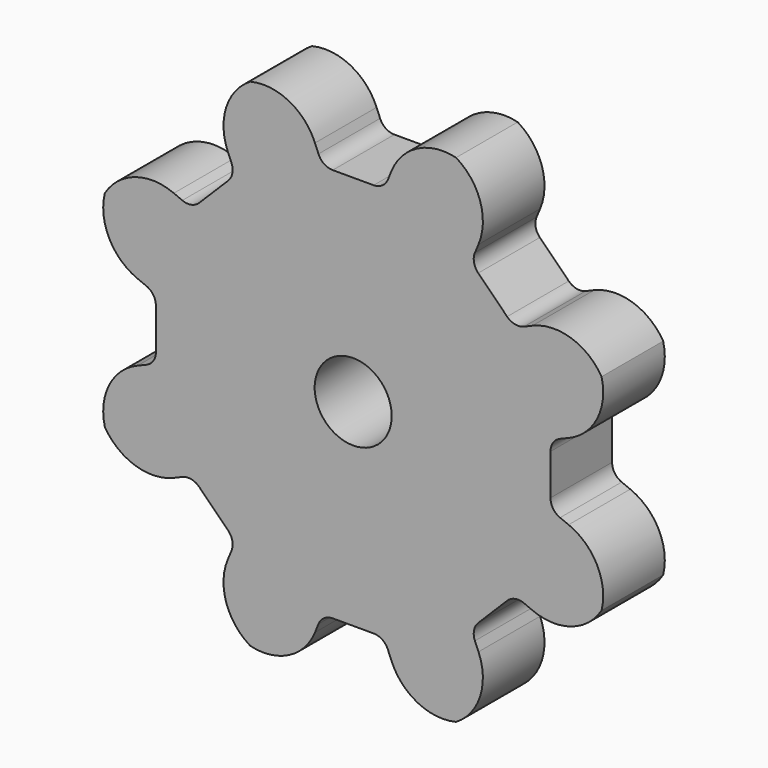
from build123d import *

# Parameters (mm, degrees)
F0_W            = 6.35
F0_H            = 22.225
F3_DEPTH        = 6.35
F3_COPIES_COUNT = 8
F4_T1_DEPTH     = 30.2839966419
F4_T3_DEPTH     = 30.283996606
F5_R            = 3.175
F6_DEPTH        = 6.35


# Not quite as in the source:
# - a fillet or chamfer that OpenCascade refuses, or shapes differently, is made with other operations: its cross-section is extruded or revolved along the edge and cut away or added
# - a pattern or mirror of a feature is missing from the dataset's text; its kind, count and spacing are read off the source's solid


with BuildPart() as f1:
    # F0 (on Right) → F1 (revolve)
    with BuildSketch(Plane.YZ):
        with Locations((3.175, 33.3375)):
            Rectangle(F0_W, F0_H)
    revolve(axis=Axis((0, 3.175, 22.225), (0, 1, 0)))

    # F2 (on Front) → F3 (cut)
    with BuildSketch(Plane.XZ):
        with BuildLine():
            Line((-1.59e-08, 38.4876703219), (-1.59e-08, 44.3230155219))
            Line((-1.59e-08, 44.3230155219), (-1.59e-08, 44.457260554))
            Line((-1.59e-08, 44.457260554), (-4.9701853855, 44.457260554))
            Line((-4.9701853855, 44.457260554), (-4.9155350159, 44.3230155219))
            Line((-4.9155350159, 44.3230155219), (-2.8620721488, 39.2788192947))
            ThreePointArc((-2.8620721488, 39.2788192947), (-2.3945935663, 38.7038580036), (-1.6858061527, 38.4876703219))
            Line((-1.6858061527, 38.4876703219), (-1.59e-08, 38.4876703219))
        make_face()
        with BuildLine():
            Line((-1.59e-08, 44.457260554), (-1.59e-08, 44.3230155219))
            Line((-1.59e-08, 44.3230155219), (-1.59e-08, 38.4876703219))
            Line((-1.59e-08, 38.4876703219), (1.6858061209, 38.4876703219))
            ThreePointArc((1.6858061209, 38.4876703219), (2.3945935345, 38.7038580036), (2.8620721171, 39.2788192947))
            Line((2.8620721171, 39.2788192947), (4.9155349841, 44.3230155219))
            Line((4.9155349841, 44.3230155219), (4.9701853538, 44.457260554))
            Line((4.9701853538, 44.457260554), (-1.59e-08, 44.457260554))
        make_face()
    f3 = extrude(amount=-F3_DEPTH, mode=Mode.SUBTRACT)

    # F3_copies: F3 ×8 about axis
    f3_copies_axis = Axis((0, 0, 22.225), (0, 1, 0))
    for i in range(1, F3_COPIES_COUNT):
        add(f3.rotate(f3_copies_axis, i * 360 / F3_COPIES_COUNT), mode=Mode.SUBTRACT)

    # F4: fillet of radius 4.572 on 16 edges, made by hand

    # F4_s2 → F4_t1 (cut)
    with BuildSketch(Plane.XZ.offset(-18.3169983209)):
        with BuildLine():
            ThreePointArc((-3.1489730441, 39.9835724397), (-5.703273274, 42.5117575675), (-9.2958119446, 42.4125829482))
            ThreePointArc((-9.2958119446, 42.4125829482), (-7.0677616426, 43.2962451071), (-4.757507246, 43.934830718))
            Line((-4.757507246, 43.934830718), (-3.1489730441, 39.9835724397))
        make_face()
        with BuildLine():
            ThreePointArc((-10.330546803, 7.4411328104), (-10.3120806372, 3.8472729487), (-7.7016451357, 1.3770915389))
            ThreePointArc((-7.7016451357, 1.3770915389), (-9.901958118, 2.3277175114), (-11.9871028839, 3.5097658457))
            Line((-11.9871028839, 3.5097658457), (-10.330546803, 7.4411328104))
        make_face()
        with BuildLine():
            ThreePointArc((3.1489730441, 4.4664275603), (5.703273274, 1.9382424325), (9.2958119446, 2.0374170518))
            ThreePointArc((9.2958119446, 2.0374170518), (7.0677616426, 1.1537548929), (4.757507246, 0.515169282))
            Line((4.757507246, 0.515169282), (3.1489730441, 4.4664275603))
        make_face()
        with BuildLine():
            ThreePointArc((14.7838671896, 11.894453197), (18.3777270513, 11.9129193628), (20.8479084611, 14.5233548643))
            ThreePointArc((20.8479084611, 14.5233548643), (19.8972824886, 12.323041882), (18.7152341543, 10.2378971161))
            Line((18.7152341543, 10.2378971161), (14.7838671896, 11.894453197))
        make_face()
        with BuildLine():
            ThreePointArc((17.7585724397, 25.3739730441), (20.2867575675, 27.928273274), (20.1875829482, 31.5208119446))
            ThreePointArc((20.1875829482, 31.5208119446), (21.0712451071, 29.2927616426), (21.709830718, 26.982507246))
            Line((21.709830718, 26.982507246), (17.7585724397, 25.3739730441))
        make_face()
        with BuildLine():
            ThreePointArc((10.330546803, 37.0088671896), (10.3120806372, 40.6027270513), (7.7016451357, 43.0729084611))
            ThreePointArc((7.7016451357, 43.0729084611), (9.901958118, 42.1222824886), (11.9871028839, 40.9402341543))
            Line((11.9871028839, 40.9402341543), (10.330546803, 37.0088671896))
        make_face()
        with BuildLine():
            ThreePointArc((-14.7838671896, 32.555546803), (-18.3777270513, 32.5370806372), (-20.8479084611, 29.9266451357))
            ThreePointArc((-20.8479084611, 29.9266451357), (-19.8972824886, 32.126958118), (-18.7152341543, 34.2121028839))
            Line((-18.7152341543, 34.2121028839), (-14.7838671896, 32.555546803))
        make_face()
        with BuildLine():
            ThreePointArc((-17.7585724397, 19.0760269559), (-20.2867575675, 16.521726726), (-20.1875829482, 12.9291880554))
            ThreePointArc((-20.1875829482, 12.9291880554), (-21.0712451071, 15.1572383574), (-21.709830718, 17.467492754))
            Line((-21.709830718, 17.467492754), (-17.7585724397, 19.0760269559))
        make_face()
    extrude(amount=F4_T1_DEPTH, mode=Mode.SUBTRACT)

    # F4_s4 → F4_t3 (cut)
    with BuildSketch(Plane.XZ.offset(-18.316998303)):
        with BuildLine():
            ThreePointArc((9.295811911, 42.4125829637), (5.7032732438, 42.5117575784), (3.1489730174, 39.983572452))
            Line((3.1489730174, 39.983572452), (4.7575072169, 43.9348307244))
            ThreePointArc((4.7575072169, 43.9348307244), (7.0677616109, 43.2962451177), (9.295811911, 42.4125829637))
        make_face()
        with BuildLine():
            ThreePointArc((-9.295811911, 2.0374170363), (-5.7032732438, 1.9382424216), (-3.1489730174, 4.466427548))
            Line((-3.1489730174, 4.466427548), (-4.7575072169, 0.5151692756))
            ThreePointArc((-4.7575072169, 0.5151692756), (-7.0677616109, 1.1537548823), (-9.295811911, 2.0374170363))
        make_face()
        with BuildLine():
            ThreePointArc((7.7016451705, 1.3770915517), (10.3120806663, 3.8472729624), (10.3305468306, 7.4411328206))
            Line((10.3305468306, 7.4411328206), (11.987102909, 3.5097658618))
            ThreePointArc((11.987102909, 3.5097658618), (9.9019581479, 2.3277175263), (7.7016451705, 1.3770915517))
        make_face()
        with BuildLine():
            ThreePointArc((20.1875829637, 12.929188089), (20.2867575784, 16.5217267562), (17.758572452, 19.0760269826))
            Line((17.758572452, 19.0760269826), (21.7098307244, 17.4674927831))
            ThreePointArc((21.7098307244, 17.4674927831), (21.0712451177, 15.1572383891), (20.1875829637, 12.929188089))
        make_face()
        with BuildLine():
            ThreePointArc((20.8479084483, 29.9266451705), (18.3777270376, 32.5370806663), (14.7838671794, 32.5555468306))
            Line((14.7838671794, 32.5555468306), (18.7152341382, 34.212102909))
            ThreePointArc((18.7152341382, 34.212102909), (19.8972824737, 32.1269581479), (20.8479084483, 29.9266451705))
        make_face()
        with BuildLine():
            ThreePointArc((-7.7016451705, 43.0729084483), (-10.3120806663, 40.6027270376), (-10.3305468306, 37.0088671794))
            Line((-10.3305468306, 37.0088671794), (-11.987102909, 40.9402341382))
            ThreePointArc((-11.987102909, 40.9402341382), (-9.9019581479, 42.1222824737), (-7.7016451705, 43.0729084483))
        make_face()
        with BuildLine():
            ThreePointArc((-20.1875829637, 31.520811911), (-20.2867575784, 27.9282732438), (-17.758572452, 25.3739730174))
            Line((-17.758572452, 25.3739730174), (-21.7098307244, 26.9825072169))
            ThreePointArc((-21.7098307244, 26.9825072169), (-21.0712451177, 29.2927616109), (-20.1875829637, 31.520811911))
        make_face()
        with BuildLine():
            ThreePointArc((-20.8479084483, 14.5233548295), (-18.3777270376, 11.9129193337), (-14.7838671794, 11.8944531694))
            Line((-14.7838671794, 11.8944531694), (-18.7152341382, 10.237897091))
            ThreePointArc((-18.7152341382, 10.237897091), (-19.8972824737, 12.3230418521), (-20.8479084483, 14.5233548295))
        make_face()
    extrude(amount=F4_T3_DEPTH, mode=Mode.SUBTRACT)

    # F5 (on Front) → F6 (cut)
    with BuildSketch(Plane.XZ):
        with Locations((0, 22.225)):
            Circle(F5_R)
    extrude(amount=-F6_DEPTH, mode=Mode.SUBTRACT)


solid = f1.part
